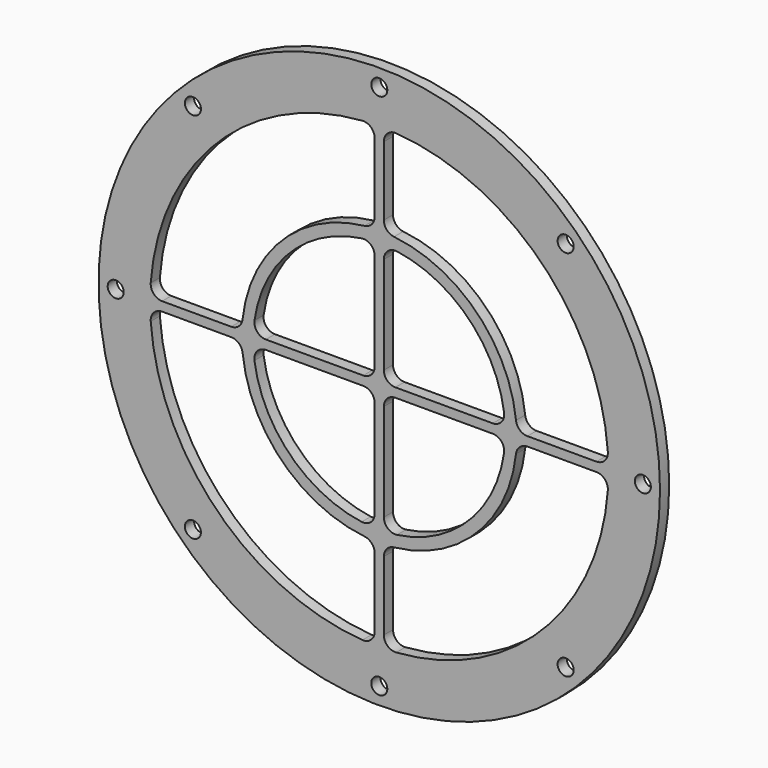
from build123d import *

# Parameters (mm, degrees)
F0_R     = 122.5
F0_R_2   = 3.5
F1_DEPTH = 5


# Not quite as in the source:
# - a feature names something its author has since deleted; it is built from what else it names


with BuildPart() as f1:
    # F0 (on Front) → F1 (new body)
    with BuildSketch(Plane.XZ):
        Circle(F0_R)
        with Locations((-81.3172798365, -81.3172798365)):
            Circle(F0_R_2, mode=Mode.SUBTRACT)
        with BuildLine():
            ThreePointArc((-99.7281623775, -7.3684210526), (-98.4052297439, -3.5972147631), (-94.7417542586, -2))
            Line((-94.7417542586, -2), (-64.6219776856, -2))
            ThreePointArc((-64.6219776856, -2), (-61.2822402478, -3.2789579623), (-59.6510563252, -6.4615384615))
            ThreePointArc((-59.6510563252, -6.4615384615), (-42.4264068712, -42.4264068712), (-6.4615384615, -59.6510563252))
            ThreePointArc((-6.4615384615, -59.6510563252), (-3.2789579623, -61.2822402478), (-2, -64.6219776856))
            Line((-2, -64.6219776856), (-2, -94.7417542586))
            ThreePointArc((-2, -94.7417542586), (-3.5972147631, -98.4052297439), (-7.3684210526, -99.7281623775))
            ThreePointArc((-7.3684210526, -99.7281623775), (-70.7106781187, -70.7106781187), (-99.7281623775, -7.3684210526))
        make_face(mode=Mode.SUBTRACT)
        with BuildLine():
            ThreePointArc((-7, -2), (-3.4644660941, -3.4644660941), (-2, -7))
            Line((-2, -7), (-2, -49.5075751779))
            ThreePointArc((-2, -49.5075751779), (-3.7212807378, -53.2824923956), (-7.7, -54.4583326957))
            ThreePointArc((-7.7, -54.4583326957), (-38.8908729653, -38.8908729653), (-54.4583326957, -7.7))
            ThreePointArc((-54.4583326957, -7.7), (-53.2824923956, -3.7212807378), (-49.5075751779, -2))
            Line((-49.5075751779, -2), (-7, -2))
        make_face(mode=Mode.SUBTRACT)
        with Locations((0, -115)):
            Circle(F0_R_2, mode=Mode.SUBTRACT)
        with Locations((81.3172798365, -81.3172798365)):
            Circle(F0_R_2, mode=Mode.SUBTRACT)
        with BuildLine():
            ThreePointArc((99.7281623775, -7.3684210526), (70.7106781187, -70.7106781187), (7.3684210526, -99.7281623775))
            ThreePointArc((7.3684210526, -99.7281623775), (3.5972147631, -98.4052297439), (2, -94.7417542586))
            Line((2, -94.7417542586), (2, -64.6219776856))
            ThreePointArc((2, -64.6219776856), (3.2789579623, -61.2822402478), (6.4615384615, -59.6510563252))
            ThreePointArc((6.4615384615, -59.6510563252), (42.4264068712, -42.4264068712), (59.6510563252, -6.4615384615))
            ThreePointArc((59.6510563252, -6.4615384615), (61.2822402478, -3.2789579623), (64.6219776856, -2))
            Line((64.6219776856, -2), (94.7417542586, -2))
            ThreePointArc((94.7417542586, -2), (98.4052297439, -3.5972147631), (99.7281623775, -7.3684210526))
        make_face(mode=Mode.SUBTRACT)
        with BuildLine():
            Line((2, -49.5075751779), (2, -7))
            ThreePointArc((2, -7), (3.4644660941, -3.4644660941), (7, -2))
            Line((7, -2), (49.5075751779, -2))
            ThreePointArc((49.5075751779, -2), (53.2824923956, -3.7212807378), (54.4583326957, -7.7))
            ThreePointArc((54.4583326957, -7.7), (38.8908729653, -38.8908729653), (7.7, -54.4583326957))
            ThreePointArc((7.7, -54.4583326957), (3.7212807378, -53.2824923956), (2, -49.5075751779))
        make_face(mode=Mode.SUBTRACT)
        with Locations((-115, 0)):
            Circle(F0_R_2, mode=Mode.SUBTRACT)
        with BuildLine():
            ThreePointArc((-2, 7), (-3.4644660941, 3.4644660941), (-7, 2))
            Line((-7, 2), (-49.5075751779, 2))
            ThreePointArc((-49.5075751779, 2), (-53.2824923956, 3.7212807378), (-54.4583326957, 7.7))
            ThreePointArc((-54.4583326957, 7.7), (-38.8908729653, 38.8908729653), (-7.7, 54.4583326957))
            ThreePointArc((-7.7, 54.4583326957), (-3.7212807378, 53.2824923956), (-2, 49.5075751779))
            Line((-2, 49.5075751779), (-2, 7))
        make_face(mode=Mode.SUBTRACT)
        with BuildLine():
            ThreePointArc((-99.7281623775, 7.3684210526), (-70.7106781187, 70.7106781187), (-7.3684210526, 99.7281623775))
            ThreePointArc((-7.3684210526, 99.7281623775), (-3.5972147631, 98.4052297439), (-2, 94.7417542586))
            Line((-2, 94.7417542586), (-2, 64.6219776856))
            ThreePointArc((-2, 64.6219776856), (-3.2789579623, 61.2822402478), (-6.4615384615, 59.6510563252))
            ThreePointArc((-6.4615384615, 59.6510563252), (-42.4264068712, 42.4264068712), (-59.6510563252, 6.4615384615))
            ThreePointArc((-59.6510563252, 6.4615384615), (-61.2822402478, 3.2789579623), (-64.6219776856, 2))
            Line((-64.6219776856, 2), (-94.7417542586, 2))
            ThreePointArc((-94.7417542586, 2), (-98.4052297439, 3.5972147631), (-99.7281623775, 7.3684210526))
        make_face(mode=Mode.SUBTRACT)
        with Locations((-81.3172798365, 81.3172798365)):
            Circle(F0_R_2, mode=Mode.SUBTRACT)
        with BuildLine():
            Line((49.5075751779, 2), (7, 2))
            ThreePointArc((7, 2), (3.4644660941, 3.4644660941), (2, 7))
            Line((2, 7), (2, 49.5075751779))
            ThreePointArc((2, 49.5075751779), (3.7212807378, 53.2824923956), (7.7, 54.4583326957))
            ThreePointArc((7.7, 54.4583326957), (38.8908729653, 38.8908729653), (54.4583326957, 7.7))
            ThreePointArc((54.4583326957, 7.7), (53.2824923956, 3.7212807378), (49.5075751779, 2))
        make_face(mode=Mode.SUBTRACT)
        with BuildLine():
            Line((2, 64.6219776856), (2, 94.7417542586))
            ThreePointArc((2, 94.7417542586), (3.5972147631, 98.4052297439), (7.3684210526, 99.7281623775))
            ThreePointArc((7.3684210526, 99.7281623775), (70.7106781187, 70.7106781187), (99.7281623775, 7.3684210526))
            ThreePointArc((99.7281623775, 7.3684210526), (98.4052297439, 3.5972147631), (94.7417542586, 2))
            Line((94.7417542586, 2), (64.6219776856, 2))
            ThreePointArc((64.6219776856, 2), (61.2822402478, 3.2789579623), (59.6510563252, 6.4615384615))
            ThreePointArc((59.6510563252, 6.4615384615), (42.4264068712, 42.4264068712), (6.4615384615, 59.6510563252))
            ThreePointArc((6.4615384615, 59.6510563252), (3.2789579623, 61.2822402478), (2, 64.6219776856))
        make_face(mode=Mode.SUBTRACT)
        with Locations((115, 0)):
            Circle(F0_R_2, mode=Mode.SUBTRACT)
        with Locations((0, 115)):
            Circle(F0_R_2, mode=Mode.SUBTRACT)
        with Locations((81.3172798365, 81.3172798365)):
            Circle(F0_R_2, mode=Mode.SUBTRACT)
    extrude(amount=F1_DEPTH)


solid = f1.part
